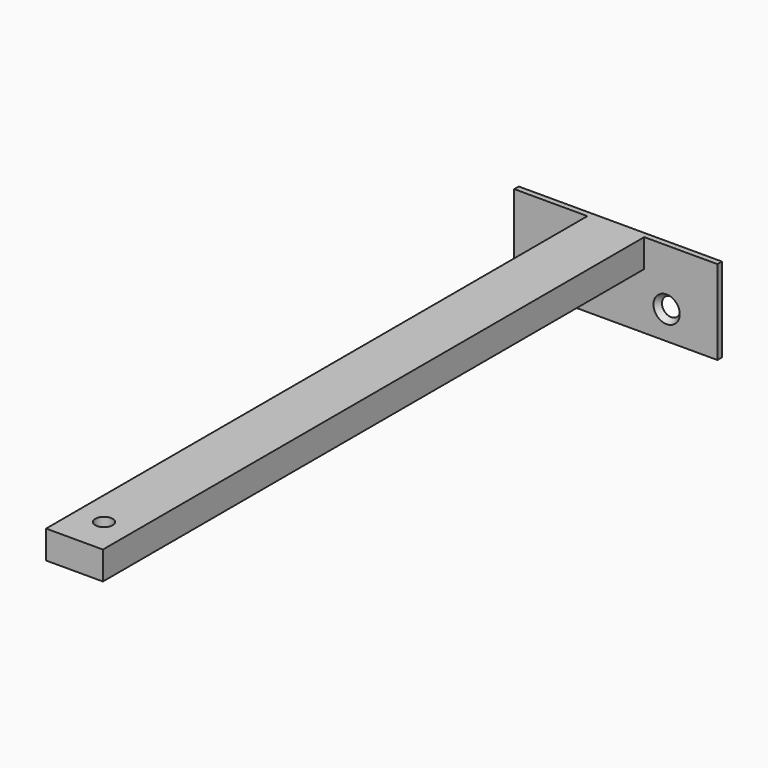
from build123d import *

# Parameters (mm, degrees)
F0_W     = 12.8171369433
F0_H     = 152.6404321194
F0_R     = 1.9711085463
F1_DEPTH = 6.35
F2_W     = 12.8171369433
F2_H     = 6.35
F2_W_2   = 16.510868445
F2_W_3   = 16.5063254535
F3_DEPTH = 1.27
F4_R     = 2.9604656486
F4_R_2   = 2.9553822982
F5_DEPTH = 1.27
F5_TAPER = 35


with BuildPart() as f1:
    # F0 (on Top) → F1 (new body)
    with BuildSketch(Plane.XY):
        Rectangle(F0_W, F0_H)
        with Locations((0, -67.9932013154)):
            Circle(F0_R, mode=Mode.SUBTRACT)
    extrude(amount=F1_DEPTH)

    # F2 (on face) → F3 (join)
    with BuildSketch(Plane(origin=(0, 76.3202160597, 0), x_dir=(-1, 0, 0), z_dir=(0, 1, 0))):
        with Locations((0, 3.175)):
            Rectangle(F2_W, F2_H)
        with Locations((-14.6640026942, 3.175)):
            Rectangle(F2_W_2, F2_H)
        with Locations((14.6617311984, 3.175)):
            Rectangle(F2_W_3, F2_H)
        Polygon((6.4085684717, 0), (-6.4085684717, 0), (-22.9194369167, 0), (-22.9194369167, -12.6968417317), (22.9148939252, -12.6968417317), (22.9148939252, 0), align=None)
    extrude(amount=F3_DEPTH)

    # F4 (on face) → F5 (cut)
    with BuildSketch(Plane.XZ.offset(-76.3202160597)):
        with Locations((11.4597184584, -6.3484208658)):
            Circle(F4_R)
        with Locations((-11.4574469626, -6.3484208658)):
            Circle(F4_R_2)
    extrude(amount=-F5_DEPTH, taper=F5_TAPER, mode=Mode.SUBTRACT)


solid = f1.part
